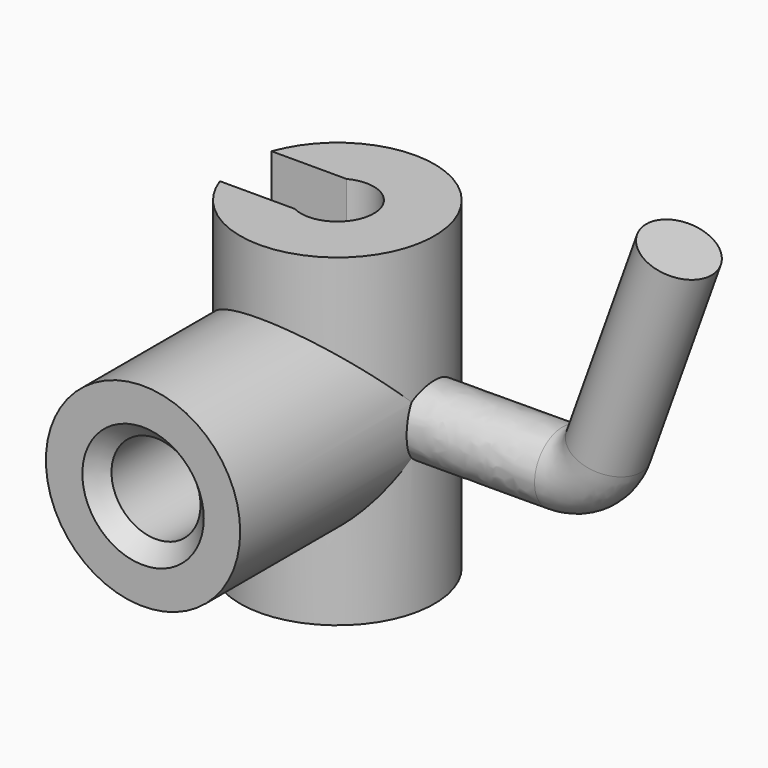
from build123d import *

# Parameters (mm, degrees)
F0_R      = 6
F1_DEPTH  = 20
F4_R      = 6
F4_R_2    = 2.75
F5_DEPTH  = 15
F7_DEPTH  = 20
F8_SIZE   = 1
F11_R     = 2.15
F2_R      = 2.25
F13_DEPTH = 20.0010001


# Not quite as in the source:
# - a feature of the source that left no trace in its solid (it failed there, or was rolled back) is left out


with BuildPart() as f1:
    # F0 (on Top) → F1 (new body)
    with BuildSketch(Plane.XY):
        Circle(F0_R)
    extrude(amount=-F1_DEPTH)

    # F4 (on offset) → F5 (join)
    with BuildSketch(Plane.XZ.offset(15)):
        with Locations((0, -10)):
            Circle(F4_R)
        with Locations((0, -10)):
            Circle(F4_R_2, mode=Mode.SUBTRACT)
    extrude(amount=-F5_DEPTH)

    # F6 (on face) → F7 (cut, through all)
    with BuildSketch(Plane.XY):
        with BuildLine():
            Line((0, 2), (-5.6568542495, 2))
            ThreePointArc((-5.6568542495, 2), (-6, 0), (-5.6568542495, -2))
            Line((-5.6568542495, -2), (0, -2))
            Line((0, -2), (0, 2))
        make_face()
        with BuildLine():
            Line((-5.6568542495, 2), (-8.5344118631, 2))
            Line((-8.5344118631, 2), (-8.5344118631, -2))
            Line((-8.5344118631, -2), (-5.6568542495, -2))
            ThreePointArc((-5.6568542495, -2), (-6, 0), (-5.6568542495, 2))
        make_face()
    extrude(amount=-F7_DEPTH, mode=Mode.SUBTRACT)

    # F8
    f8_edges = [f1.edges().sort_by_distance(p)[0] for p in [
        (-2.75, -15, -10),
    ]]
    chamfer(f8_edges, length=F8_SIZE)

    # F12: sweep along a path in F10
    with BuildLine(Plane.XZ) as f12_path:
        Line((0, -10), (13.8992802655, -9.9480403702))
        ThreePointArc((13.8992802655, -9.9480403702), (15.6179693755, -9.3990677428), (16.7109593102, -7.9635761178))
        Line((16.7109593102, -7.9635761178), (21.0774621296, 4.1742816034))
    # F11 (on offset) → F12 (sweep)
    with BuildSketch(Plane.YZ.offset(6)):
        with Locations((0, -10)):
            Circle(F11_R)
    sweep(path=f12_path.line)

    # F2 (on face) → F13 (cut, through all)
    with BuildSketch(Plane.XY):
        Circle(F2_R)
    extrude(amount=-F13_DEPTH, mode=Mode.SUBTRACT)


solid = f1.part
